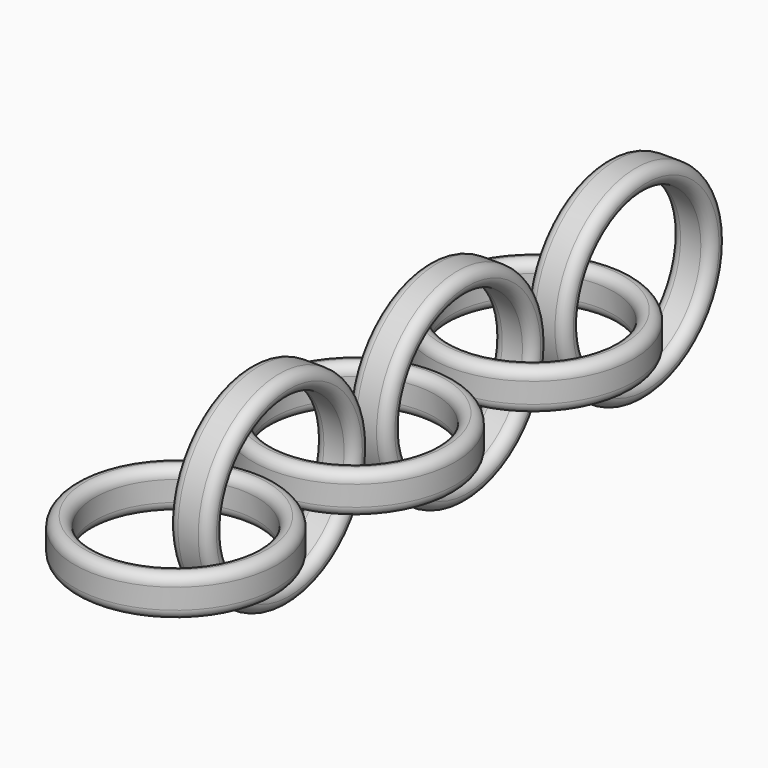
from build123d import *

# Parameters (mm, degrees)
F0_R     = 10
F0_R_2   = 8
F1_DEPTH = 2
F2_R     = 0.99999
F5_R     = 10
F5_R_2   = 8
F6_DEPTH = 2
F7_R     = 0.99999


# Not quite as in the source:
# - a fillet or chamfer is up to 0.001 mm smaller than in the source, because OpenCascade refuses the exact size


with BuildPart() as f1:
    # F0 (on Top) → F1 (new body, symmetric)
    with BuildSketch(Plane.XY):
        Circle(F0_R)
        Circle(F0_R_2, mode=Mode.SUBTRACT)
    extrude(amount=F1_DEPTH, both=True)

    # F2 (radius 1 in the source; OpenCascade refuses exactly that, so slightly less here)
    f2_edges = [f1.edges().sort_by_distance(p)[0] for p in [
        (-10, 0, 2),
        (-8, 0, 2),
        (-10, 0, -2),
        (-8, 0, -2),
    ]]
    fillet(f2_edges, radius=F2_R)


with BuildPart() as f3_1:
    # F3: copy of F1
    add(f1.part.moved(Location((0, 22, 0))))


with BuildPart() as f4_1:
    # F4: copy of F1
    add(f1.part.moved(Location((0, -22, 0))))


with BuildPart() as f6:
    # F5 (on Right) → F6 (new body, symmetric)
    with BuildSketch(Plane.YZ):
        with Locations((-10.4954766127, 0)):
            Circle(F5_R)
        with Locations((-10.4954766127, 0)):
            Circle(F5_R_2, mode=Mode.SUBTRACT)
    extrude(amount=F6_DEPTH, both=True)

    # F7 (radius 1 in the source; OpenCascade refuses exactly that, so slightly less here)
    f7_edges = [f6.edges().sort_by_distance(p)[0] for p in [
        (-2, -18.495477, 0),
        (2, -18.495477, 0),
        (-2, -20.495477, 0),
        (2, -20.495477, 0),
    ]]
    fillet(f7_edges, radius=F7_R)


with BuildPart() as f8_1:
    # F8: copy of F6
    add(f6.part.moved(Location((0, 22, 0))))


with BuildPart() as f9_1:
    # F9: copy of F8_1
    add(f8_1.part.moved(Location((0, 22, 0))))


solid = Compound([f1.part, f3_1.part, f4_1.part, f6.part, f8_1.part, f9_1.part])
